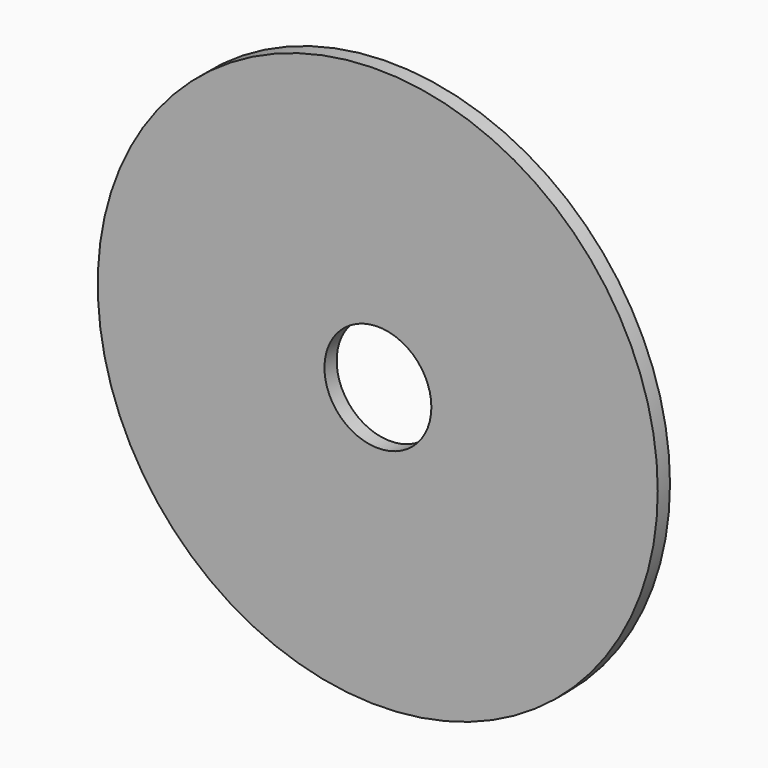
from build123d import *

# Parameters (mm, degrees)
F0_R     = 10.668
F1_DEPTH = 3.048


# Not quite as in the source:
# - a feature names something its author has since deleted; it is built from what else it names


with BuildPart() as f1:
    # F0 (on Front) → F1 (new body)
    with BuildSketch(Plane.XZ):
        with BuildLine():
            ThreePointArc((-40.259899137, 38.7519666788), (-20.8908022371, -51.8280694401), (55.88, 0))
            ThreePointArc((55.88, 0), (51.824470852, 20.8997277713), (40.2465490009, 38.7658315211))
            ThreePointArc((40.2465490009, 38.7658315211), (-0.0096236685, 55.8799991713), (-40.259899137, 38.7519666788))
        make_face()
        with Locations((0.0326246152, 0.0217348816)):
            Circle(F0_R, mode=Mode.SUBTRACT)
    extrude(amount=F1_DEPTH)


solid = f1.part
